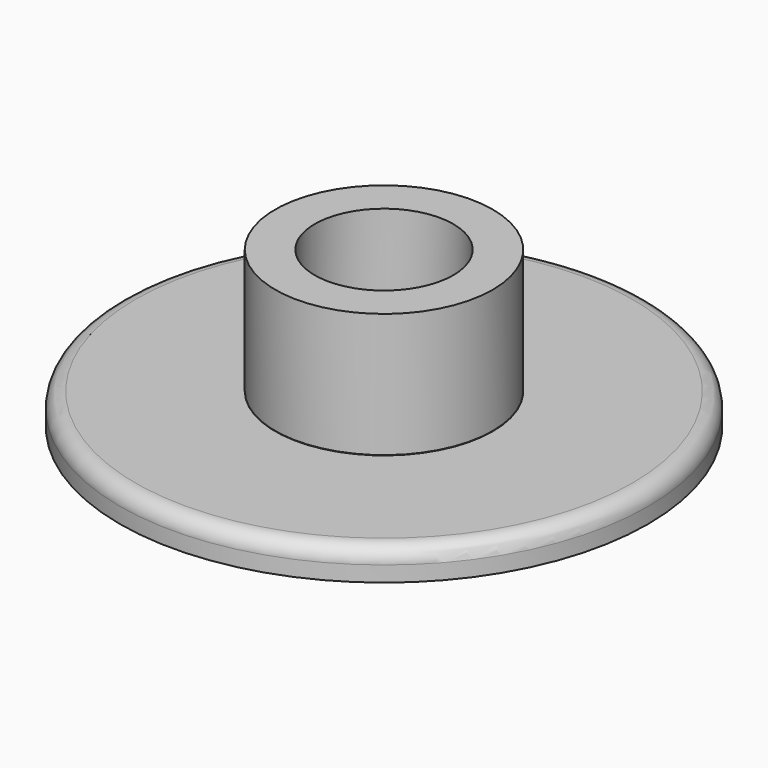
from build123d import *

# Parameters (mm, degrees)
F0_R     = 3.5
F1_DEPTH = 4
F0_R_2   = 8.5
F2_DEPTH = 1
F3_R     = 0.5
F4_T     = -1.27


# Not quite as in the source:
# - a fillet or chamfer that OpenCascade refuses, or shapes differently, is made with other operations: its cross-section is extruded or revolved along the edge and cut away or added


with BuildPart() as f1:
    # F0 (on Top) → F1 (new body)
    with BuildSketch(Plane.XY):
        Circle(F0_R)
    extrude(amount=F1_DEPTH)

    # F4
    f4_openings = [f1.faces().sort_by_distance(p)[0] for p in [
        (0, 0, 4),
    ]]
    offset(amount=F4_T, openings=f4_openings)


with BuildPart() as f2:
    # F0 (on Top) → F2 (new body)
    with BuildSketch(Plane.XY):
        Circle(F0_R_2)
        Circle(F0_R, mode=Mode.SUBTRACT)
    extrude(amount=F2_DEPTH)

    # F3
    f3_edges = [f2.edges().sort_by_distance(p)[0] for p in [
        (-8.5, 0, 1),
    ]]
    fillet(f3_edges, radius=F3_R)


with BuildPart() as f2_1:
    # F5: moved
    add(f2.part.moved(Location((0, 0, -1.0112))))

    # F6: fillet of radius 11.8962787499 on 1 edges, made by hand

    # F6_s1 → F6_t2 (revolve, cut)
    with BuildSketch(Plane.XZ):
        with BuildLine():
            ThreePointArc((8.2741551609, -1.0112), (5.8352743981, -0.7585164303), (3.5, -0.0112))
            Line((3.5, -0.0112), (3.4045168968, -0.229125575))
            ThreePointArc((3.4045168968, -0.229125575), (3.262074425, -0.5112), (3.262074425, -1.0112))
            Line((3.262074425, -1.0112), (3.5, -1.249125575))
            Line((3.5, -1.249125575), (8.2741551609, -1.249125575))
            Line((8.2741551609, -1.249125575), (8.2741551609, -1.0112))
        make_face()
    revolve(axis=Axis((0, 0, -1.0112), (0, 0, 1)), mode=Mode.SUBTRACT)


solid = Compound([f1.part, f2_1.part])
